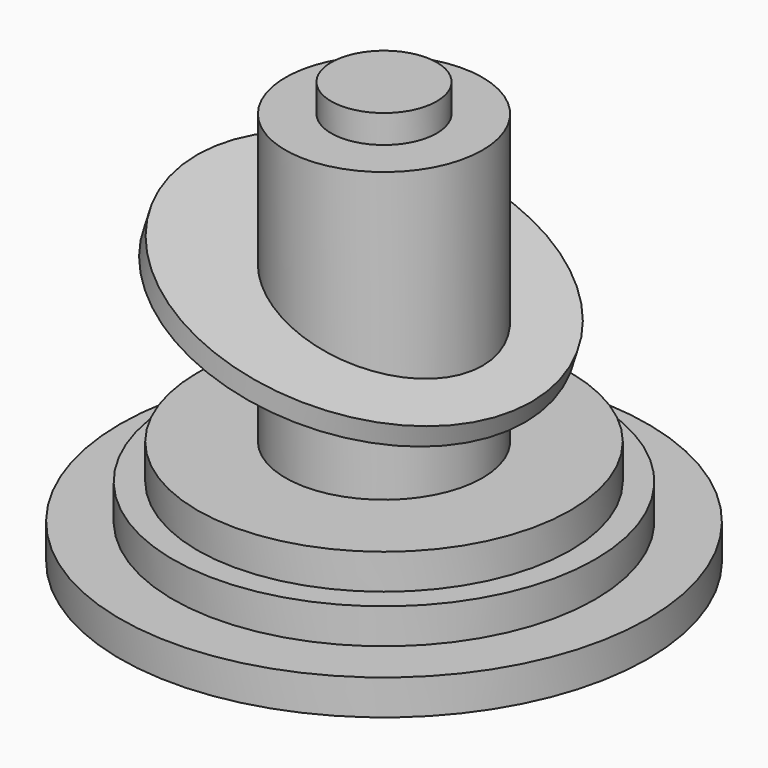
from build123d import *

# Parameters (mm, degrees)
F0_W      = 2
F0_H      = 2
F1_DEPTH  = 1
F2_R      = 7.5
F3_DEPTH  = 60
F4_R      = 14
F5_DEPTH  = 56
F6_R      = 37.5
F7_DEPTH  = 5
F8_R      = 30
F9_DEPTH  = 10
F10_R     = 26.5
F11_DEPTH = 15
F12_R     = 25
F13_DEPTH = 3
F14_ANGLE = 18


with BuildPart() as f1:
    # F0 (on Front) → F1 (new body, symmetric)
    with BuildSketch(Plane.XZ):
        Rectangle(F0_W, F0_H)
    extrude(amount=F1_DEPTH, both=True)


with BuildPart() as f3:
    # F2 (on Top) → F3 (new body)
    with BuildSketch(Plane.XY):
        Circle(F2_R)
    extrude(amount=F3_DEPTH)

    # F4 (on Top) → F5 (join)
    with BuildSketch(Plane.XY):
        Circle(F4_R)
    extrude(amount=F5_DEPTH)

    # F6 (on Top) → F7 (join)
    with BuildSketch(Plane.XY):
        Circle(F6_R)
    extrude(amount=F7_DEPTH)

    # F8 (on Top) → F9 (join)
    with BuildSketch(Plane.XY):
        Circle(F8_R)
    extrude(amount=F9_DEPTH)

    # F10 (on Top) → F11 (join)
    with BuildSketch(Plane.XY):
        Circle(F10_R)
    extrude(amount=F11_DEPTH)


with BuildPart() as f13:
    # F12 (on Top) → F13 (new body)
    with BuildSketch(Plane.XY):
        Circle(F12_R)
    extrude(amount=F13_DEPTH)


with BuildPart() as f13_1:
    # F14: moved
    add(f13.part.rotate(Axis((-1, 0, -1), (0, 1, 0)), F14_ANGLE))


with BuildPart() as f13_2:
    # F15: moved
    add(f13_1.part.moved(Location((-4, 0, 32))))


solid = Compound([f1.part, f3.part, f13_2.part])
